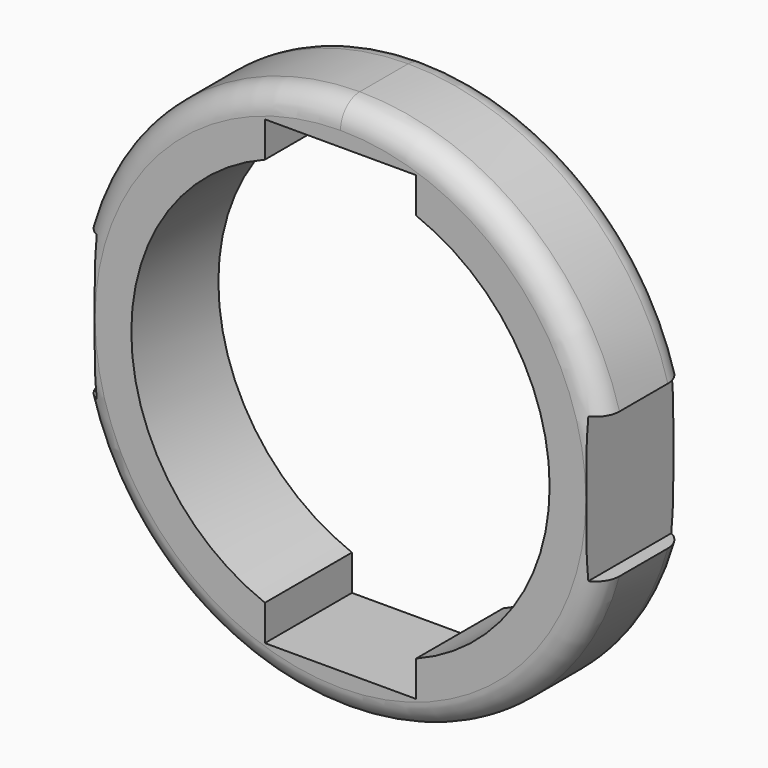
from build123d import *

# Parameters (mm, degrees)
F0_R          = 8.65
F1_DEPTH      = 2.25
F1_DEPTH_BACK = 2.25
F2_R          = 1
F3_W          = 6.250812
F3_H          = 19.070166
F3_W_2        = 1.701653
F3_H_2        = 6
F4_DEPTH      = 25
F4_DEPTH_BACK = 25


with BuildPart() as f1:
    # F0 (on Front) → F1 (new body, two sides)
    with BuildSketch(Plane.XZ) as f1_sk:
        with BuildLine():
            ThreePointArc((-11.15, 0), (0, -11.15), (11.15, 0))
            ThreePointArc((11.15, 0), (7.884241, 7.884241), (0, 11.15))
            ThreePointArc((0, 11.15), (-7.884241, 7.884241), (-11.15, 0))
        make_face()
        Circle(F0_R, mode=Mode.SUBTRACT)
    extrude(amount=F1_DEPTH)
    extrude(f1_sk.sketch, amount=-F1_DEPTH_BACK)

    # F2
    f2_edges = [f1.edges().sort_by_distance(p)[0] for p in [
        (-11.15, -2.25, 0),
        (-11.15, 2.25, 0),
    ]]
    fillet(f2_edges, radius=F2_R)

    # F3 (on Front) → F4 (cut, two sides)
    with BuildSketch(Plane.XZ) as f4_sk:
        Rectangle(F3_W, F3_H)
        with Locations((11.015831, 0)):
            Rectangle(F3_W_2, F3_H_2)
        with Locations((-11.015831, 0)):
            Rectangle(F3_W_2, F3_H_2)
    extrude(amount=F4_DEPTH, mode=Mode.SUBTRACT)
    extrude(f4_sk.sketch, amount=-F4_DEPTH_BACK, mode=Mode.SUBTRACT)


solid = f1.part
